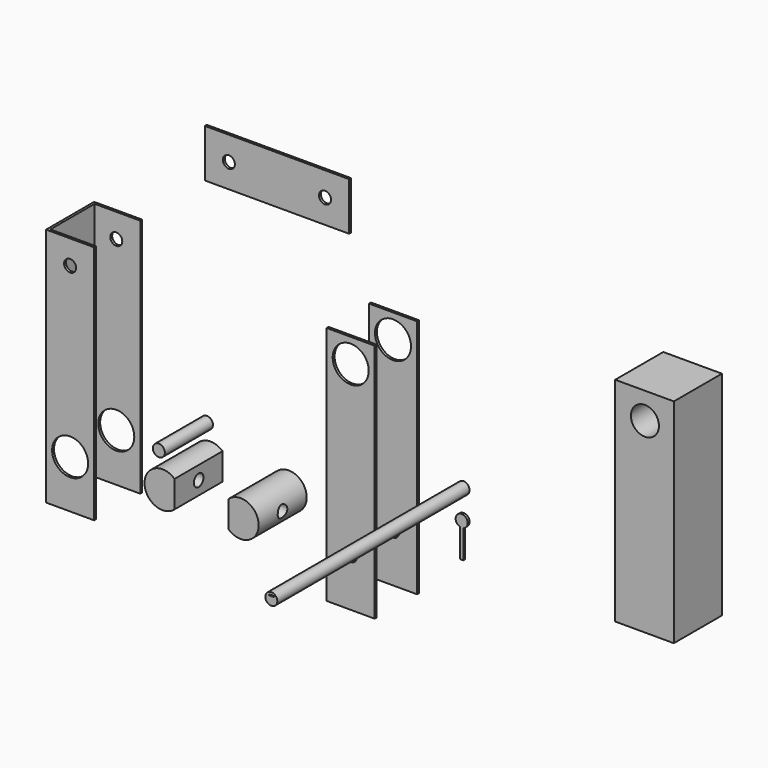
from build123d import *

# Parameters (mm, degrees)
F0_W      = 20
F0_H      = 100
F0_R      = 7.5
F0_R_2    = 2.5
F1_DEPTH  = 25
F2_DEPTH  = 25
F3_W      = 19
F3_H      = 23
F4_DEPTH  = 100
F5_DEPTH  = 23
F6_W      = 19
F6_H      = 21
F7_DEPTH  = 100
F8_W      = 23
F8_H      = 40
F9_DEPTH  = 1
F10_W     = 21
F10_H     = 40
F11_DEPTH = 1
F12_DEPTH = 25
F13_R     = 2.5
F14_DEPTH = 12.5
F15_DEPTH = 25
F16_R     = 2.5
F17_DEPTH = 12.5010001006
F18_DEPTH = 100
F19_DEPTH = 1
F20_W     = 1.9876025617
F20_H     = 0.3975201398
F21_DEPTH = 2
F22_W     = 0.4727318883
F22_H     = 1.4182012528
F22_W_2   = 0.4216358066
F22_H_2   = 1.0189469904
F23_DEPTH = 2
F0_W_2    = 60
F0_H_2    = 20
F24_DEPTH = 1
F0_W_3    = 24.4019627571
F0_H_3    = 88.5824598372
F0_R_3    = 5.8378194673
F25_DEPTH = 25
F26_T     = -2.5


with BuildPart() as f1:
    # F0 (on Front) → F1 (new body)
    with BuildSketch(Plane.XZ):
        with Locations((-85.3658488447, -19.1779926979)):
            Rectangle(F0_W, F0_H)
        with Locations((-85.3658488447, -49.1779926979)):
            Circle(F0_R, mode=Mode.SUBTRACT)
        with Locations((-85.3658488447, 20.8220073021)):
            Circle(F0_R_2, mode=Mode.SUBTRACT)
    extrude(amount=F1_DEPTH)

    # F3 (on face) → F4 (cut)
    with BuildSketch(Plane(origin=(0, 0, -69.1779926979), x_dir=(1, 0, 0), z_dir=(0, 0, -1))):
        with Locations((-84.8658488447, 12.5)):
            Rectangle(F3_W, F3_H)
    extrude(amount=-F4_DEPTH, mode=Mode.SUBTRACT)

    # F8 (on face) → F9 (cut, through all)
    with BuildSketch(Plane(origin=(-95.3658488447, 0, 0), x_dir=(0, -1, 0), z_dir=(-1, 0, 0))):
        with Locations((12.5, -49.1779926979)):
            Rectangle(F8_W, F8_H)
    extrude(amount=-F9_DEPTH, mode=Mode.SUBTRACT)


with BuildPart() as f2:
    # F0 (on Front) → F2 (new body)
    with BuildSketch(Plane.XZ):
        with Locations((-48.4434533864, -34.8060615361)):
            Circle(F0_R_2)
    extrude(amount=F2_DEPTH)


with BuildPart() as f5:
    # F0 (on Front) → F5 (new body)
    with BuildSketch(Plane.XZ):
        with Locations((29.7814775258, -18.581676666)):
            Rectangle(F0_W, F0_H)
        with Locations((29.7814775258, -48.581676666)):
            Circle(F0_R_2, mode=Mode.SUBTRACT)
        with Locations((29.7814775258, 21.418323334)):
            Circle(F0_R, mode=Mode.SUBTRACT)
    extrude(amount=F5_DEPTH)

    # F6 (on face) → F7 (cut)
    with BuildSketch(Plane(origin=(0, 0, -68.581676666), x_dir=(1, 0, 0), z_dir=(0, 0, -1))):
        with Locations((30.2814775258, 11.5)):
            Rectangle(F6_W, F6_H)
    extrude(amount=-F7_DEPTH, mode=Mode.SUBTRACT)

    # F10 (on face) → F11 (cut, through all)
    with BuildSketch(Plane(origin=(19.7814775258, 0, 0), x_dir=(0, -1, 0), z_dir=(-1, 0, 0))):
        with Locations((11.5, 11.418323334)):
            Rectangle(F10_W, F10_H)
    extrude(amount=-F11_DEPTH, mode=Mode.SUBTRACT)


with BuildPart() as f12:
    # F0 (on Front) → F12 (new body)
    with BuildSketch(Plane.XZ):
        with BuildLine():
            Line((-41.9182138266, -54.3014750868), (-41.9182138266, -43.1211351993))
            ThreePointArc((-41.9182138266, -43.1211351993), (-54.4182138266, -48.7113051431), (-41.9182138266, -54.3014750868))
        make_face()
    extrude(amount=F12_DEPTH)

    # F13 (on face) → F14 (cut, through all)
    with BuildSketch(Plane.YZ.offset(-41.9182138266)):
        with Locations((-12.4340476468, -48.7113051431)):
            Circle(F13_R)
    extrude(amount=-F14_DEPTH, mode=Mode.SUBTRACT)


with BuildPart() as f15:
    # F0 (on Front) → F15 (new body)
    with BuildSketch(Plane.XZ):
        with BuildLine():
            ThreePointArc((-19.4155542431, -54.3014750868), (-6.9155542431, -48.7113051431), (-19.4155542431, -43.1211351993))
            Line((-19.4155542431, -43.1211351993), (-19.4155542431, -54.3014750868))
        make_face()
    extrude(amount=F15_DEPTH)

    # F16 (on face) → F17 (cut, through all)
    with BuildSketch(Plane(origin=(-19.4155542431, 0, 0), x_dir=(0, -1, 0), z_dir=(-1, 0, 0))):
        with Locations((12.5784268603, -48.7897321582)):
            Circle(F16_R)
    extrude(amount=-F17_DEPTH, mode=Mode.SUBTRACT)


with BuildPart() as f18:
    # F0 (on Front) → F18 (new body)
    with BuildSketch(Plane.XZ):
        with Locations((58.3449043334, -24.0014214069)):
            Circle(F0_R_2)
    extrude(amount=F18_DEPTH)

    # F20 (on face) → F21 (cut)
    with BuildSketch(Plane.XZ.offset(100)):
        with Locations((58.4452617913, -22.7724621072)):
            Rectangle(F20_W, F20_H)
    extrude(amount=-F21_DEPTH, mode=Mode.SUBTRACT)

    # F22 (on face) → F23 (cut)
    with BuildSketch(Plane.XZ):
        with Locations((59.7926527262, -23.7945998088)):
            Rectangle(F22_W, F22_H)
        with Locations((57.0760257542, -23.5474118963)):
            Rectangle(F22_W_2, F22_H_2)
    extrude(amount=F23_DEPTH, mode=Mode.SUBTRACT)


with BuildPart() as f19:
    # F0 (on Front) → F19 (new body)
    with BuildSketch(Plane.XZ):
        with BuildLine():
            Line((59.0452197349, -49.8900748789), (59.0452197349, -38.0256086664))
            ThreePointArc((59.0452197349, -38.0256086664), (58.3449043334, -33.125700681), (57.6445889318, -38.0256086664))
            Line((57.6445889318, -38.0256086664), (57.6445889318, -49.8900748789))
            Line((57.6445889318, -49.8900748789), (58.3449043334, -49.8900748789))
            Line((58.3449043334, -49.8900748789), (59.0452197349, -49.8900748789))
        make_face()
    extrude(amount=F19_DEPTH)


with BuildPart() as f24:
    # F0 (on Front) → F24 (new body)
    with BuildSketch(Plane.XZ):
        with Locations((-18.5069639981, 64.2900748551)):
            Rectangle(F0_W_2, F0_H_2)
        with Locations((-38.5069639981, 64.2900748551)):
            Circle(F0_R_2, mode=Mode.SUBTRACT)
        with Locations((1.4930360019, 64.2900748551)):
            Circle(F0_R_2, mode=Mode.SUBTRACT)
    extrude(amount=F24_DEPTH)


with BuildPart() as f25:
    # F0 (on Front) → F25 (new body)
    with BuildSketch(Plane.XZ):
        with Locations((153.6454260349, 8.5435975343)):
            Rectangle(F0_W_3, F0_H_3)
        with Locations((153.81257236, 41.8038032949)):
            Circle(F0_R_3, mode=Mode.SUBTRACT)
    extrude(amount=F25_DEPTH)

    # F26
    f26_openings = [f25.faces().sort_by_distance(p)[0] for p in [
        (141.444445, -12.5, 8.543598),
    ]]
    offset(amount=F26_T, openings=f26_openings)


solid = Compound([f1.part, f2.part, f5.part, f12.part, f15.part, f18.part, f19.part, f24.part, f25.part])
